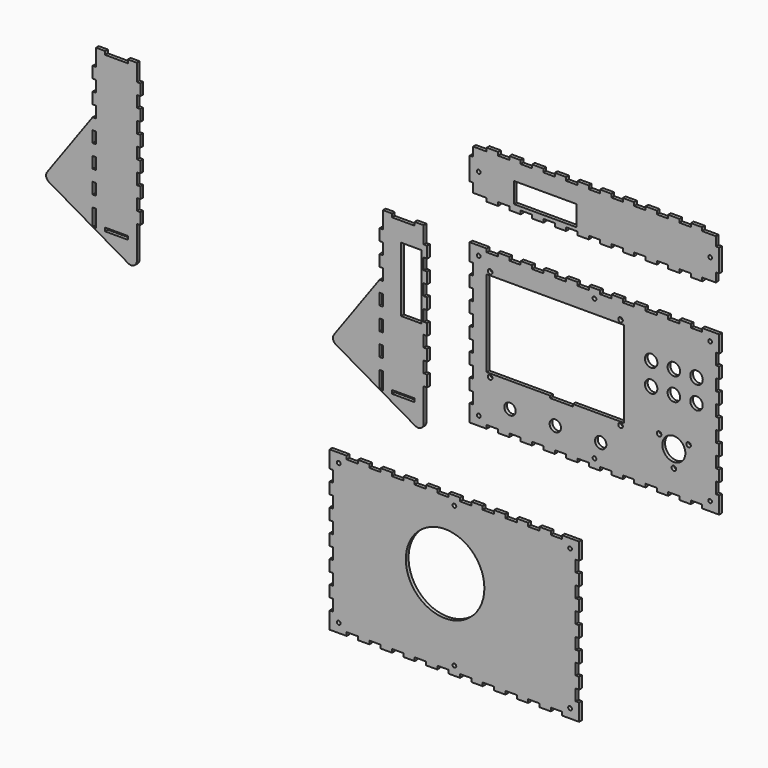
from build123d import *

# Parameters (mm, degrees)
F0_R     = 1.65
F0_R_2   = 5
F0_R_3   = 2
F0_R_4   = 10.15
F0_R_5   = 5.5
F2_DEPTH = 3
F0_W     = 20
F0_H     = 3
F0_W_2   = 3
F0_H_2   = 10
F0_W_3   = 18
F0_H_3   = 57
F0_R_6   = 34.6359322433
F0_W_4   = 55
F0_H_4   = 18


# Not quite as in the source:
# - a feature of the source that left no trace in its solid (it failed there, or was rolled back) is left out


with BuildPart() as f2:
    # F0 (on Front) → F2 (new body)
    with BuildSketch(Plane.XZ):
        Polygon((-75.5, -67), (-75.5, -82), (-60.5, -82), (-60.5, -79), (-50.5, -79), (-50.5, -82), (-40.5, -82), (-40.5, -79), (-30.5, -79), (-30.5, -82), (-20.5, -82), (-20.5, -79), (-10.5, -79), (-10.5, -82), (-0.5, -82), (-0.5, -79), (9.5, -79), (9.5, -82), (19.5, -82), (19.5, -79), (29.5, -79), (29.5, -82), (39.5, -82), (39.5, -79), (49.5, -79), (49.5, -82), (59.5, -82), (59.5, -79), (69.5, -79), (69.5, -82), (79.5, -82), (79.5, -79), (89.5, -79), (89.5, -82), (99.5, -82), (99.5, -79), (109.5, -79), (109.5, -82), (119.5, -82), (119.5, -79), (129.5, -79), (129.5, -82), (144.5, -82), (144.5, -79), (144.5, -67), (141.5, -67), (141.5, -57), (144.5, -57), (144.5, -47), (141.5, -47), (141.5, -37), (144.5, -37), (144.5, -27), (141.5, -27), (141.5, -17), (144.5, -17), (144.5, -7), (141.5, -7), (141.5, 3), (144.5, 3), (144.5, 13), (141.5, 13), (141.5, 23), (144.5, 23), (144.5, 33), (141.5, 33), (141.5, 43), (144.5, 43), (144.5, 55), (144.5, 58), (129.5, 58), (129.5, 55), (119.5, 55), (119.5, 58), (109.5, 58), (109.5, 55), (99.5, 55), (99.5, 58), (89.5, 58), (89.5, 55), (79.5, 55), (79.5, 58), (69.5, 58), (69.5, 55), (59.5, 55), (59.5, 58), (49.5, 58), (49.5, 55), (39.5, 55), (39.5, 58), (29.5, 58), (29.5, 55), (19.5, 55), (19.5, 58), (9.5, 58), (9.5, 55), (-0.5, 55), (-0.5, 58), (-10.5, 58), (-10.5, 55), (-20.5, 55), (-20.5, 58), (-30.5, 58), (-30.5, 55), (-40.5, 55), (-40.5, 58), (-50.5, 58), (-50.5, 55), (-60.5, 55), (-60.5, 58), (-75.5, 58), (-75.5, 43), (-72.5, 43), (-72.5, 33), (-75.5, 33), (-75.5, 23), (-72.5, 23), (-72.5, 13), (-75.5, 13), (-75.5, 3), (-72.5, 3), (-72.5, -7), (-75.5, -7), (-75.5, -17), (-72.5, -17), (-72.5, -27), (-75.5, -27), (-75.5, -37), (-72.5, -37), (-72.5, -47), (-75.5, -47), (-75.5, -57), (-72.5, -57), (-72.5, -67), align=None)
        with Locations((-67.5, -74)):
            Circle(F0_R, mode=Mode.SUBTRACT)
        with Locations((34.5, -74)):
            Circle(F0_R, mode=Mode.SUBTRACT)
        with Locations((136.5, -74)):
            Circle(F0_R, mode=Mode.SUBTRACT)
        with Locations((-40, -60)):
            Circle(F0_R_2, mode=Mode.SUBTRACT)
        with Locations((-57.5, -41)):
            Circle(F0_R_3, mode=Mode.SUBTRACT)
        with Locations((0, -60)):
            Circle(F0_R_2, mode=Mode.SUBTRACT)
        with Locations((40, -60)):
            Circle(F0_R_2, mode=Mode.SUBTRACT)
        with Locations((57.5, -41)):
            Circle(F0_R_3, mode=Mode.SUBTRACT)
        with Locations((104.5, -59)):
            Circle(F0_R_3, mode=Mode.SUBTRACT)
        with Locations((104.5, -44)):
            Circle(F0_R_4, mode=Mode.SUBTRACT)
        with Locations((91.5096189432, -36.5)):
            Circle(F0_R_3, mode=Mode.SUBTRACT)
        with Locations((117.4903810568, -36.5)):
            Circle(F0_R_3, mode=Mode.SUBTRACT)
        Polygon((-60.5, -38), (-60.5, 38), (60.5, 38), (60.5, -38), (15.5, -38), (15.5, -40), (-4.5, -40), (-4.5, -38), align=None, mode=Mode.SUBTRACT)
        with Locations((84.5, -2)):
            Circle(F0_R_5, mode=Mode.SUBTRACT)
        with Locations((104.5, -2)):
            Circle(F0_R_5, mode=Mode.SUBTRACT)
        with Locations((124.5, -2)):
            Circle(F0_R_5, mode=Mode.SUBTRACT)
        with Locations((84.5, 18)):
            Circle(F0_R_5, mode=Mode.SUBTRACT)
        with Locations((104.5, 18)):
            Circle(F0_R_5, mode=Mode.SUBTRACT)
        with Locations((124.5, 18)):
            Circle(F0_R_5, mode=Mode.SUBTRACT)
        with Locations((-57.5, 41)):
            Circle(F0_R_3, mode=Mode.SUBTRACT)
        with Locations((-67.5, 50)):
            Circle(F0_R, mode=Mode.SUBTRACT)
        with Locations((57.5, 41)):
            Circle(F0_R_3, mode=Mode.SUBTRACT)
        with Locations((34.5, 50)):
            Circle(F0_R, mode=Mode.SUBTRACT)
        with Locations((136.5, 50)):
            Circle(F0_R, mode=Mode.SUBTRACT)
    extrude(amount=F2_DEPTH)


with BuildPart() as f2b:
    # F0 (on Front) → F2, piece 2 (new body)
    with BuildSketch(Plane.XZ):
        with BuildLine():
            Line((-116.037769556, 43), (-116.037769556, 58))
            Line((-116.037769556, 58), (-124.037769556, 58))
            Line((-124.037769556, 58), (-124.037769556, 55))
            Line((-124.037769556, 55), (-144.037769556, 55))
            Line((-144.037769556, 55), (-144.037769556, 58))
            Line((-144.037769556, 58), (-152.037769556, 58))
            Line((-152.037769556, 58), (-152.037769556, 43))
            Line((-152.037769556, 43), (-155.037769556, 43))
            Line((-155.037769556, 43), (-155.037769556, 33))
            Line((-155.037769556, 33), (-152.037769556, 33))
            Line((-152.037769556, 33), (-152.037769556, 23))
            Line((-152.037769556, 23), (-155.037769556, 23))
            Line((-155.037769556, 23), (-155.037769556, 13))
            Line((-155.037769556, 13), (-152.037769556, 13))
            Line((-152.037769556, 13), (-152.037769556, 3))
            Line((-152.037769556, 3), (-155.037769556, 3))
            Line((-155.037769556, 3), (-195.099743843, -52.5114999333))
            ThreePointArc((-195.099743843, -52.5114999333), (-195.9343959947, -56.4848737041), (-193.5453195726, -59.7676556321))
            Line((-193.5453195726, -59.7676556321), (-155.037769556, -82))
            Line((-155.037769556, -82), (-123.537769556, -100.1865334795))
            ThreePointArc((-123.537769556, -100.1865334795), (-118.537769556, -100.1865334795), (-116.037769556, -95.8564064606))
            Line((-116.037769556, -95.8564064606), (-116.037769556, -82))
            Line((-116.037769556, -82), (-116.037769556, -67))
            Line((-116.037769556, -67), (-113.037769556, -67))
            Line((-113.037769556, -67), (-113.037769556, -57))
            Line((-113.037769556, -57), (-116.037769556, -57))
            Line((-116.037769556, -57), (-116.037769556, -47))
            Line((-116.037769556, -47), (-113.037769556, -47))
            Line((-113.037769556, -47), (-113.037769556, -37))
            Line((-113.037769556, -37), (-116.037769556, -37))
            Line((-116.037769556, -37), (-116.037769556, -27))
            Line((-116.037769556, -27), (-113.037769556, -27))
            Line((-113.037769556, -27), (-113.037769556, -17))
            Line((-113.037769556, -17), (-116.037769556, -17))
            Line((-116.037769556, -17), (-116.037769556, -7))
            Line((-116.037769556, -7), (-113.037769556, -7))
            Line((-113.037769556, -7), (-113.037769556, 3))
            Line((-113.037769556, 3), (-116.037769556, 3))
            Line((-116.037769556, 3), (-116.037769556, 13))
            Line((-116.037769556, 13), (-113.037769556, 13))
            Line((-113.037769556, 13), (-113.037769556, 23))
            Line((-113.037769556, 23), (-116.037769556, 23))
            Line((-116.037769556, 23), (-116.037769556, 33))
            Line((-116.037769556, 33), (-113.037769556, 33))
            Line((-113.037769556, 33), (-113.037769556, 43))
            Line((-113.037769556, 43), (-116.037769556, 43))
        make_face()
        with BuildLine():
            Line((-155.037769556, -81.99), (-155.037769556, -67))
            Line((-155.037769556, -67), (-152.037769556, -67))
            Line((-152.037769556, -67), (-152.037769556, -82))
            Line((-152.037769556, -82), (-155.027769556, -82))
            ThreePointArc((-155.027769556, -82), (-155.0348406239, -81.9970710678), (-155.037769556, -81.99))
        make_face(mode=Mode.SUBTRACT)
        with Locations((-134.037769556, -80.5)):
            Rectangle(F0_W, F0_H, mode=Mode.SUBTRACT)
        with Locations((-153.537769556, -52)):
            Rectangle(F0_W_2, F0_H_2, mode=Mode.SUBTRACT)
        with Locations((-153.537769556, -32)):
            Rectangle(F0_W_2, F0_H_2, mode=Mode.SUBTRACT)
        with Locations((-153.537769556, -12)):
            Rectangle(F0_W_2, F0_H_2, mode=Mode.SUBTRACT)
        with Locations((-127.037769556, 9.5)):
            Rectangle(F0_W_3, F0_H_3, mode=Mode.SUBTRACT)
    extrude(amount=F2_DEPTH)


with BuildPart() as f2c:
    # F0 (on Front) → F2, piece 3 (new body)
    with BuildSketch(Plane.XZ):
        with BuildLine():
            Line((-369.0009684563, 86.8499703846), (-369.0009684563, 101.8499703846))
            Line((-369.0009684563, 101.8499703846), (-377.0009684563, 101.8499703846))
            Line((-377.0009684563, 101.8499703846), (-377.0009684563, 98.8499703846))
            Line((-377.0009684563, 98.8499703846), (-397.0009684563, 98.8499703846))
            Line((-397.0009684563, 98.8499703846), (-397.0009684563, 101.8499703846))
            Line((-397.0009684563, 101.8499703846), (-405.0009684563, 101.8499703846))
            Line((-405.0009684563, 101.8499703846), (-405.0009684563, 86.8499703846))
            Line((-405.0009684563, 86.8499703846), (-408.0009684563, 86.8499703846))
            Line((-408.0009684563, 86.8499703846), (-408.0009684563, 76.8499703846))
            Line((-408.0009684563, 76.8499703846), (-405.0009684563, 76.8499703846))
            Line((-405.0009684563, 76.8499703846), (-405.0009684563, 66.8499703846))
            Line((-405.0009684563, 66.8499703846), (-408.0009684563, 66.8499703846))
            Line((-408.0009684563, 66.8499703846), (-408.0009684563, 56.8499703846))
            Line((-408.0009684563, 56.8499703846), (-405.0009684563, 56.8499703846))
            Line((-405.0009684563, 56.8499703846), (-405.0009684563, 46.8499703846))
            Line((-405.0009684563, 46.8499703846), (-408.0442427657, 46.8499703846))
            Line((-408.0442427657, 46.8499703846), (-448.1062170527, -8.6615295486))
            ThreePointArc((-448.1062170527, -8.6615295486), (-448.9408692043, -12.6349033195), (-446.5517927823, -15.9176852474))
            Line((-446.5517927823, -15.9176852474), (-408.0442427657, -38.1500296154))
            Line((-408.0442427657, -38.1500296154), (-376.5009684563, -56.361547529))
            ThreePointArc((-376.5009684563, -56.361547529), (-371.5009684563, -56.361547529), (-369.0009684563, -52.0314205101))
            Line((-369.0009684563, -52.0314205101), (-369.0009684563, -38.1500296154))
            Line((-369.0009684563, -38.1500296154), (-369.0009684563, -23.1500296154))
            Line((-369.0009684563, -23.1500296154), (-366.0009684563, -23.1500296154))
            Line((-366.0009684563, -23.1500296154), (-366.0009684563, -13.1500296154))
            Line((-366.0009684563, -13.1500296154), (-369.0009684563, -13.1500296154))
            Line((-369.0009684563, -13.1500296154), (-369.0009684563, -3.1500296154))
            Line((-369.0009684563, -3.1500296154), (-366.0009684563, -3.1500296154))
            Line((-366.0009684563, -3.1500296154), (-366.0009684563, 6.8499703846))
            Line((-366.0009684563, 6.8499703846), (-369.0009684563, 6.8499703846))
            Line((-369.0009684563, 6.8499703846), (-369.0009684563, 16.8499703846))
            Line((-369.0009684563, 16.8499703846), (-366.0009684563, 16.8499703846))
            Line((-366.0009684563, 16.8499703846), (-366.0009684563, 26.8499703846))
            Line((-366.0009684563, 26.8499703846), (-369.0009684563, 26.8499703846))
            Line((-369.0009684563, 26.8499703846), (-369.0009684563, 36.8499703846))
            Line((-369.0009684563, 36.8499703846), (-366.0009684563, 36.8499703846))
            Line((-366.0009684563, 36.8499703846), (-366.0009684563, 46.8499703846))
            Line((-366.0009684563, 46.8499703846), (-369.0009684563, 46.8499703846))
            Line((-369.0009684563, 46.8499703846), (-369.0009684563, 56.8499703846))
            Line((-369.0009684563, 56.8499703846), (-366.0009684563, 56.8499703846))
            Line((-366.0009684563, 56.8499703846), (-366.0009684563, 66.8499703846))
            Line((-366.0009684563, 66.8499703846), (-369.0009684563, 66.8499703846))
            Line((-369.0009684563, 66.8499703846), (-369.0009684563, 76.8499703846))
            Line((-369.0009684563, 76.8499703846), (-366.0009684563, 76.8499703846))
            Line((-366.0009684563, 76.8499703846), (-366.0009684563, 86.8499703846))
            Line((-366.0009684563, 86.8499703846), (-369.0009684563, 86.8499703846))
        make_face()
        with Locations((-387.0009684563, -36.6500296154)):
            Rectangle(F0_W, F0_H, mode=Mode.SUBTRACT)
        with BuildLine():
            Line((-408.0442427657, -38.1400296154), (-408.0442427657, -23.1500296154))
            Line((-408.0442427657, -23.1500296154), (-405.0009684563, -23.1500296154))
            Line((-405.0009684563, -23.1500296154), (-405.0009684563, -38.1500296154))
            Line((-405.0009684563, -38.1500296154), (-408.0342427657, -38.1500296154))
            ThreePointArc((-408.0342427657, -38.1500296154), (-408.0413138335, -38.1471006832), (-408.0442427657, -38.1400296154))
        make_face(mode=Mode.SUBTRACT)
        with Locations((-406.5009684563, -8.1500296154)):
            Rectangle(F0_W_2, F0_H_2, mode=Mode.SUBTRACT)
        with Locations((-406.5009684563, 11.8499703846)):
            Rectangle(F0_W_2, F0_H_2, mode=Mode.SUBTRACT)
        with Locations((-406.5009684563, 31.8499703846)):
            Rectangle(F0_W_2, F0_H_2, mode=Mode.SUBTRACT)
    extrude(amount=F2_DEPTH)


with BuildPart() as f2d:
    # F0 (on Front) → F2, piece 4 (new body)
    with BuildSketch(Plane.XZ):
        Polygon((-184, -142.9839320272), (-199, -142.9839320272), (-199, -157.9839320272), (-196, -157.9839320272), (-196, -167.9839320272), (-199, -167.9839320272), (-199, -177.9839320272), (-196, -177.9839320272), (-196, -187.9839320272), (-199, -187.9839320272), (-199, -197.9839320272), (-196, -197.9839320272), (-196, -207.9839320272), (-199, -207.9839320272), (-199, -217.9839320272), (-196, -217.9839320272), (-196, -227.9839320272), (-199, -227.9839320272), (-199, -237.9839320272), (-196, -237.9839320272), (-196, -247.9839320272), (-199, -247.9839320272), (-199, -257.9839320272), (-196, -257.9839320272), (-196, -267.9839320272), (-199, -267.9839320272), (-199, -282.9839320272), (-194, -282.9839320272), (-184, -282.9839320272), (-184, -279.9839320272), (-174, -279.9839320272), (-174, -282.9839320272), (-164, -282.9839320272), (-164, -279.9839320272), (-154, -279.9839320272), (-154, -282.9839320272), (-144, -282.9839320272), (-144, -279.9839320272), (-134, -279.9839320272), (-134, -282.9839320272), (-124, -282.9839320272), (-124, -279.9839320272), (-114, -279.9839320272), (-114, -282.9839320272), (-104, -282.9839320272), (-104, -279.9839320272), (-94, -279.9839320272), (-94, -282.9839320272), (-84, -282.9839320272), (-84, -279.9839320272), (-74, -279.9839320272), (-74, -282.9839320272), (-64, -282.9839320272), (-64, -279.9839320272), (-54, -279.9839320272), (-54, -282.9839320272), (-44, -282.9839320272), (-44, -279.9839320272), (-34, -279.9839320272), (-34, -282.9839320272), (-24, -282.9839320272), (-24, -279.9839320272), (-14, -279.9839320272), (-14, -282.9839320272), (-4, -282.9839320272), (-4, -279.9839320272), (6, -279.9839320272), (6, -282.9839320272), (11, -282.9839320272), (21, -282.9839320272), (21, -267.9839320272), (18, -267.9839320272), (18, -257.9839320272), (21, -257.9839320272), (21, -247.9839320272), (18, -247.9839320272), (18, -237.9839320272), (21, -237.9839320272), (21.0067172812, -227.9839342833), (18, -227.9839342833), (18, -217.9839342833), (21, -217.9839342833), (21, -207.9839342833), (18, -207.9839342833), (18, -197.9839342833), (21, -197.9839342833), (21, -187.9839342833), (18, -187.9839342833), (18, -177.9839342833), (21, -177.9839342833), (21, -167.9839342833), (18, -167.9839342833), (18, -157.9839342833), (21, -157.9839342833), (21, -145.9839320272), (21, -142.9839320272), (6, -142.9839320272), (6, -145.9839320272), (-4, -145.9839320272), (-4, -142.9839320272), (-14, -142.9839320272), (-14, -145.9839320272), (-24, -145.9839320272), (-24, -142.9839320272), (-34, -142.9839320272), (-34, -145.9839320272), (-44, -145.9839320272), (-44, -142.9839320272), (-54, -142.9839320272), (-54, -145.9839320272), (-64, -145.9839320272), (-64, -142.9839320272), (-74, -142.9839320272), (-74, -145.9839320272), (-84, -145.9839320272), (-84, -142.9839320272), (-94, -142.9839320272), (-94, -145.9839320272), (-104, -145.9839320272), (-104, -142.9839320272), (-114, -142.9839320272), (-114, -145.9839320272), (-124, -145.9839320272), (-124, -142.9839320272), (-134, -142.9839320272), (-134, -145.9839320272), (-144, -145.9839320272), (-144, -142.9839320272), (-154, -142.9839320272), (-154, -145.9839320272), (-164, -145.9839320272), (-164, -142.9839320272), (-174, -142.9839320272), (-174, -145.9839320272), (-184, -145.9839320272), align=None)
        with Locations((-191, -274.9839320272)):
            Circle(F0_R, mode=Mode.SUBTRACT)
        with Locations((-191, -150.9839320272)):
            Circle(F0_R, mode=Mode.SUBTRACT)
        with Locations((-89, -274.9839320272)):
            Circle(F0_R, mode=Mode.SUBTRACT)
        with Locations((-97.1954092383, -206.4019888639)):
            Circle(F0_R_6, mode=Mode.SUBTRACT)
        with Locations((13, -274.9839320272)):
            Circle(F0_R, mode=Mode.SUBTRACT)
        with Locations((-89, -150.9839320272)):
            Circle(F0_R, mode=Mode.SUBTRACT)
        with Locations((13, -150.9839320272)):
            Circle(F0_R, mode=Mode.SUBTRACT)
    extrude(amount=F2_DEPTH)


with BuildPart() as f2e:
    # F0 (on Front) → F2, piece 5 (new body)
    with BuildSketch(Plane.XZ):
        Polygon((-60.5, 97.2545017004), (-60.5, 94.2545017004), (-50.5, 94.2545017004), (-50.5, 97.2545017004), (-40.5, 97.2545017004), (-40.5, 94.2545017004), (-30.5, 94.2545017004), (-30.5, 97.2545017004), (-20.5, 97.2545017004), (-20.5, 94.2545017004), (-10.5, 94.2545017004), (-10.5, 97.2545017004), (-0.5, 97.2545017004), (-0.5, 94.2545017004), (9.5, 94.2545017004), (9.5, 97.2545017004), (19.5, 97.2545017004), (19.5, 94.2545017004), (29.5, 94.2545017004), (29.5, 97.2545017004), (39.5, 97.2545017004), (39.5, 94.2545017004), (49.5, 94.2545017004), (49.5, 97.2545017004), (59.5, 97.2545017004), (59.5, 94.2545017004), (69.5, 94.2545017004), (69.5, 97.2545017004), (79.5, 97.2545017004), (79.5, 94.2545017004), (89.5, 94.2545017004), (89.5, 97.2545017004), (99.5, 97.2545017004), (99.5, 94.2545017004), (109.5, 94.2545017004), (109.5, 97.2545017004), (119.5, 97.2545017004), (119.5, 94.2545017004), (129.5, 94.2545017004), (129.5, 97.2545017004), (139.5, 97.2545017004), (141.5, 97.2545017004), (141.5, 105.2545017004), (144.5, 105.2545017004), (144.5, 125.2545017004), (141.5, 125.2545017004), (141.5, 133.2545017004), (139.5, 133.2545017004), (129.5, 133.2545017004), (129.5, 136.2545017004), (119.5, 136.2545017004), (119.5, 133.2545017004), (109.5, 133.2545017004), (109.5, 136.2545017004), (99.5, 136.2545017004), (99.5, 133.2545017004), (89.5, 133.2545017004), (89.5, 136.2545017004), (79.5, 136.2545017004), (79.5, 133.2545017004), (69.5, 133.2545017004), (69.5, 136.2545017004), (59.5, 136.2545017004), (59.5, 133.2545017004), (49.5, 133.2545017004), (49.5, 136.2545017004), (39.5, 136.2545017004), (39.5, 133.2545017004), (29.5, 133.2545017004), (29.5, 136.2545017004), (19.5, 136.2545017004), (19.5, 133.2545017004), (9.5, 133.2545017004), (9.5, 136.2545017004), (-0.5, 136.2545017004), (-0.5, 133.2545017004), (-10.5, 133.2545017004), (-10.5, 136.2545017004), (-20.5, 136.2545017004), (-20.5, 133.2545017004), (-30.5, 133.2545017004), (-30.5, 136.2545017004), (-40.5, 136.2545017004), (-40.5, 133.2545017004), (-50.5, 133.2545017004), (-50.5, 136.2545017004), (-60.5, 136.2545017004), (-60.5, 133.2545017004), (-72.5, 133.2545017004), (-72.5, 125.2545017004), (-75.5, 125.2545017004), (-75.5, 105.2545017004), (-72.5, 105.2545017004), (-72.5, 97.2545017004), align=None)
        with Locations((-9, 109.2545017004)):
            Rectangle(F0_W_4, F0_H_4, mode=Mode.SUBTRACT)
        with Locations((-67.5, 115.2545017004)):
            Circle(F0_R, mode=Mode.SUBTRACT)
        with Locations((136.5, 115.2545017004)):
            Circle(F0_R, mode=Mode.SUBTRACT)
    extrude(amount=F2_DEPTH)


solid = Compound([f2.part, f2b.part, f2c.part, f2d.part, f2e.part])
